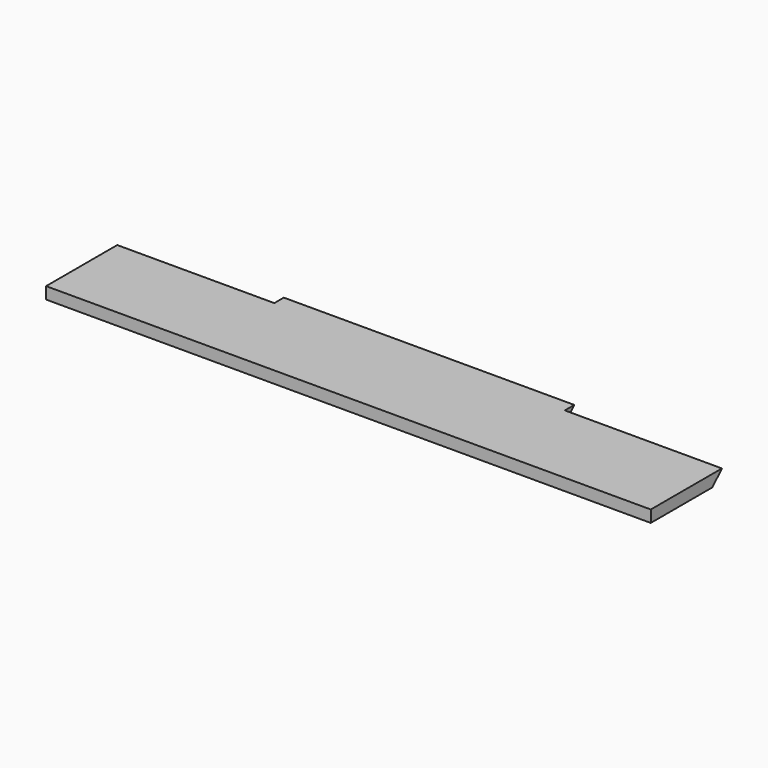
from build123d import *

# Parameters (mm, degrees)
F1_DEPTH = 4
F2_SIZE  = 3.99999
F3_SIZE  = 3.99999
F4_SIZE  = 3.99999


# Not quite as in the source:
# - a fillet or chamfer is up to 0.001 mm smaller than in the source, because OpenCascade refuses the exact size


with BuildPart() as f1:
    # F0 (on Top) → F1 (new body)
    with BuildSketch(Plane.XY):
        Polygon((-102, 0), (0, 0), (102, 0), (102, 30), (49, 30), (49, 34), (-49, 34), (-49, 30), (-102, 30), align=None)
    extrude(amount=F1_DEPTH)

    # F2 (size 4 in the source; OpenCascade refuses exactly that, so slightly less here)
    f2_edges = [f1.edges().sort_by_distance(p)[0] for p in [
        (75.5, 30, 0),
    ]]
    chamfer(f2_edges, length=F2_SIZE)

    # F3 (size 4 in the source; OpenCascade refuses exactly that, so slightly less here)
    f3_edges = [f1.edges().sort_by_distance(p)[0] for p in [
        (0, 34, 0),
    ]]
    chamfer(f3_edges, length=F3_SIZE)

    # F4 (size 4 in the source; OpenCascade refuses exactly that, so slightly less here)
    f4_edges = [f1.edges().sort_by_distance(p)[0] for p in [
        (-75.5, 30, 0),
    ]]
    chamfer(f4_edges, length=F4_SIZE)


solid = f1.part
